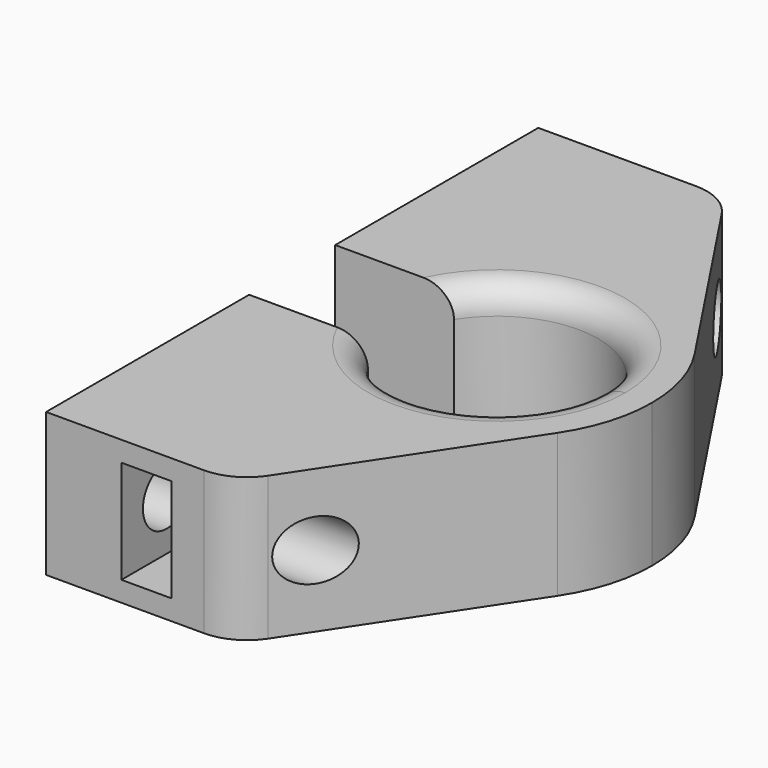
from build123d import *

# Parameters (mm, degrees)
F3_DEPTH = 8
F4_DEPTH = 1
F5_R     = 1.65
F6_DEPTH = 13.5965032877
F9_DEPTH = 2.8
F10_R    = 1.5
F11_R    = 3


# Not quite as in the source:
# - a pattern or mirror of a feature is missing from the dataset's text; its kind, count and spacing are read off the source's solid
# - a feature names something its author has since deleted; it is built from what else it names


with BuildPart() as f3:
    # F2 (on Top) → F3 (new body)
    with BuildSketch(Plane.XY):
        with BuildLine():
            Line((-11.41, 3), (-8.1131066799, 3))
            ThreePointArc((-8.1131066799, 3), (-0.999988831, 8.5920033949), (7.2072655829, 4.7830767104))
            Line((7.2072655829, 4.7830767104), (-1, 17.15))
            Line((-1, 17.15), (-11.41, 17.15))
            Line((-11.41, 17.15), (-11.41, 3))
        make_face()
        with BuildLine():
            ThreePointArc((7.2072655829, -4.7830767104), (-0.999988831, -8.5920033949), (-8.1131066799, -3))
            Line((-8.1131066799, -3), (-11.41, -3))
            Line((-11.41, -3), (-11.41, -17.15))
            Line((-11.41, -17.15), (-1, -17.15))
            Line((-1, -17.15), (7.2072655829, -4.7830767104))
        make_face()
        with BuildLine():
            ThreePointArc((-4.7877447718, 3), (1.5607277212, 5.430159204), (5.65, 0))
            ThreePointArc((5.65, 0), (1.5607277212, -5.430159204), (-4.7877447718, -3))
            Line((-4.7877447718, -3), (-8.1131066799, -3))
            ThreePointArc((-8.1131066799, -3), (-0.999988831, -8.5920033949), (7.2072655829, -4.7830767104))
            ThreePointArc((7.2072655829, -4.7830767104), (8.2814656702, -2.4979644421), (8.65, 0))
            ThreePointArc((8.65, 0), (8.2814656702, 2.4979644421), (7.2072655829, 4.7830767104))
            ThreePointArc((7.2072655829, 4.7830767104), (-0.999988831, 8.5920033949), (-8.1131066799, 3))
            Line((-8.1131066799, 3), (-4.7877447718, 3))
        make_face()
    extrude(amount=F3_DEPTH)

    # F2 (on Top) → F4 (join)
    with BuildSketch(Plane.XY):
        with BuildLine():
            ThreePointArc((-4.7877447718, -3), (1.5607277212, -5.430159204), (5.65, 0))
            ThreePointArc((5.65, 0), (1.5607277212, 5.430159204), (-4.7877447718, 3))
            Line((-4.7877447718, 3), (-3.9373214245, 3))
            ThreePointArc((-3.9373214245, 3), (1.5831549117, 4.6900021882), (4.95, 0))
            ThreePointArc((4.95, 0), (1.5831549117, -4.6900021882), (-3.9373214245, -3))
            Line((-3.9373214245, -3), (-4.7877447718, -3))
        make_face()
    extrude(amount=F4_DEPTH)

    # F5 (on face) → F6 (cut, through all)
    with BuildSketch(Plane(origin=(-11.41, 0, 0), x_dir=(0, -1, 0), z_dir=(-1, 0, 0))):
        with Locations((14, 4)):
            Circle(F5_R)
        with Locations((-14, 4)):
            Circle(F5_R)
    extrude(amount=-F6_DEPTH, mode=Mode.SUBTRACT)

    # F8 (on offset) → F9 (cut)
    with BuildSketch(Plane(origin=(-7.21, 0, 0), x_dir=(0, -1, 0), z_dir=(-1, 0, 0))):
        Polygon((17.15, 6.875), (15.6598820239, 6.875), (17.15, 4.2940399562), align=None)
        Polygon((17.15, 4.2940399562), (15.6598820239, 6.875), (12.3401179761, 6.875), (10.6802359522, 4), (12.3401179761, 1.125), (15.6598820239, 1.125), (17.15, 3.7059600438), align=None)
        Polygon((17.3197640478, 4), (17.15, 4.2940399562), (17.15, 3.7059600438), align=None)
        Polygon((17.15, 1.125), (17.15, 3.7059600438), (15.6598820239, 1.125), align=None)
    f9 = extrude(amount=-F9_DEPTH, mode=Mode.SUBTRACT)

    # F9_copies: F9 across plane
    add(f9.mirror(Plane.ZX), mode=Mode.SUBTRACT)

    # F10
    f10_edges = [f3.edges().sort_by_distance(p)[0] for p in [
        (5.65, 0, 8),
    ]]
    fillet(f10_edges, radius=F10_R)

    # F11
    f11_edges = [f3.edges().sort_by_distance(p)[0] for p in [
        (-1, -17.15, 4),
        (-1, 17.15, 4),
    ]]
    fillet(f11_edges, radius=F11_R)


solid = f3.part
